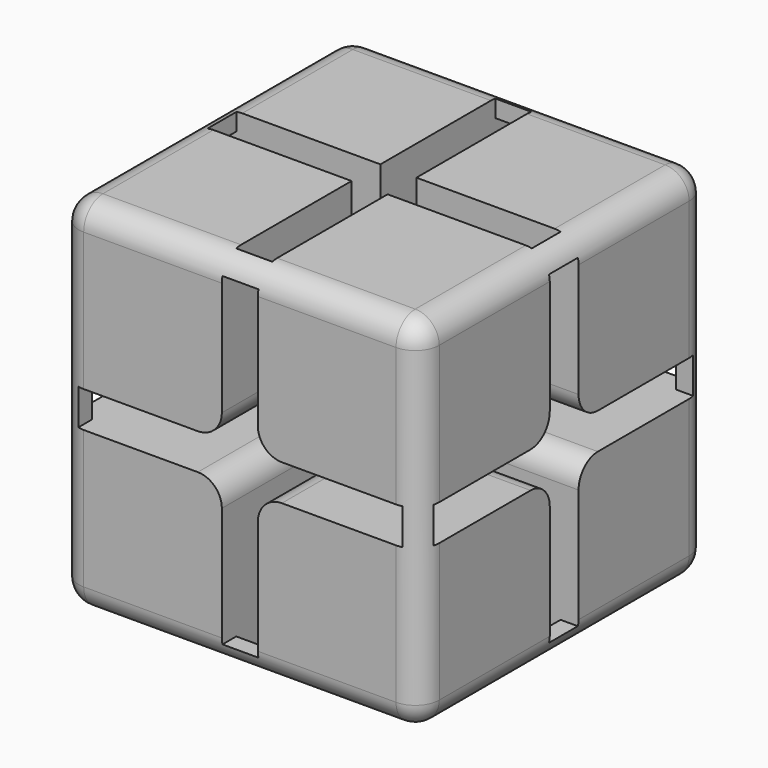
from build123d import *

# Parameters (mm, degrees)
F0_W         = 76.2
F0_H         = 76.2
F1_DEPTH     = 76.2
F3_DEPTH     = 76.2
F5_DEPTH     = 76.2
F7_DEPTH     = 76.2
F8_T1_DEPTH  = 66.04
F8_T3_DEPTH  = 66.04
F8_T5_DEPTH  = 66.04
F8_S9_W      = 5.08
F8_S9_H      = 5.08
F8_T10_DEPTH = 5.08
F8_S15_W     = 5.08
F8_S15_H     = 5.08
F8_T16_DEPTH = 5.08
F8_S21_W     = 5.08
F8_S21_H     = 5.08
F8_T22_DEPTH = 5.08
F8_S27_W     = 5.08
F8_S27_H     = 5.08
F8_T28_DEPTH = 5.08
F8_S33_W     = 5.08
F8_S33_H     = 5.08
F8_T34_DEPTH = 5.08
F8_S39_W     = 5.08
F8_S39_H     = 5.08
F8_T40_DEPTH = 5.08
F8_S45_W     = 5.08
F8_S45_H     = 5.08
F8_T46_DEPTH = 5.08
F8_S51_W     = 5.08
F8_S51_H     = 5.08
F8_T52_DEPTH = 5.08
F9_R         = 5.08


# Not quite as in the source:
# - a fillet or chamfer that OpenCascade refuses, or shapes differently, is made with other operations: its cross-section is extruded or revolved along the edge and cut away or added


with BuildPart() as f1:
    # F0 (on Top) → F1 (new body)
    with BuildSketch(Plane.XY):
        Rectangle(F0_W, F0_H)
    extrude(amount=F1_DEPTH)

    # F2 (on face) → F3 (cut)
    with BuildSketch(Plane.XZ.offset(38.1)):
        Polygon((-3.81, 41.91), (-34.29, 41.91), (-34.29, 34.29), (-3.81, 34.29), (-3.81, 3.81), (3.81, 3.81), (3.81, 34.29), (34.29, 34.29), (34.29, 41.91), (3.81, 41.91), (3.81, 72.39), (-3.81, 72.39), align=None)
    extrude(amount=-F3_DEPTH, mode=Mode.SUBTRACT)

    # F4 (on face) → F5 (cut)
    with BuildSketch(Plane.XY.offset(76.2)):
        Polygon((3.81, 34.29), (-3.81, 34.29), (-3.81, 3.81), (-34.29, 3.81), (-34.29, -3.81), (-3.81, -3.81), (-3.81, -34.29), (3.81, -34.29), (3.81, -3.81), (34.29, -3.81), (34.29, 3.81), (3.81, 3.81), align=None)
    extrude(amount=-F5_DEPTH, mode=Mode.SUBTRACT)

    # F6 (on face) → F7 (cut)
    with BuildSketch(Plane.YZ.offset(38.1)):
        Polygon((-3.81, 41.91), (-34.29, 41.91), (-34.29, 34.29), (-3.81, 34.29), (-3.81, 3.81), (3.81, 3.81), (3.81, 34.29), (34.29, 34.29), (34.29, 41.91), (3.81, 41.91), (3.81, 72.39), (-3.81, 72.39), align=None)
    extrude(amount=-F7_DEPTH, mode=Mode.SUBTRACT)

    # F8: fillet of radius 5.08 on 12 edges, made by hand

    # F8_s2 → F8_t1 (cut)
    with BuildSketch(Plane.XY.offset(5.08)):
        with BuildLine():
            ThreePointArc((33.02, -38.1), (36.6121024484, -36.6121024484), (38.1, -33.02))
            Line((38.1, -33.02), (38.1, -38.1))
            Line((38.1, -38.1), (33.02, -38.1))
        make_face()
        with BuildLine():
            ThreePointArc((-33.02, -38.1), (-36.6121024484, -36.6121024484), (-38.1, -33.02))
            Line((-38.1, -33.02), (-38.1, -38.1))
            Line((-38.1, -38.1), (-33.02, -38.1))
        make_face()
        with BuildLine():
            ThreePointArc((33.02, 38.1), (36.6121024484, 36.6121024484), (38.1, 33.02))
            Line((38.1, 33.02), (38.1, 38.1))
            Line((38.1, 38.1), (33.02, 38.1))
        make_face()
        with BuildLine():
            ThreePointArc((-33.02, 38.1), (-36.6121024484, 36.6121024484), (-38.1, 33.02))
            Line((-38.1, 33.02), (-38.1, 38.1))
            Line((-38.1, 38.1), (-33.02, 38.1))
        make_face()
    extrude(amount=F8_T1_DEPTH, mode=Mode.SUBTRACT)

    # F8_s4 → F8_t3 (cut)
    with BuildSketch(Plane.YZ.offset(-33.02)):
        with BuildLine():
            ThreePointArc((-38.1, 71.12), (-36.6121024484, 74.7121024484), (-33.02, 76.2))
            Line((-33.02, 76.2), (-38.1, 76.2))
            Line((-38.1, 76.2), (-38.1, 71.12))
        make_face()
        with BuildLine():
            ThreePointArc((-38.1, 5.08), (-36.6121024484, 1.4878975516), (-33.02, 0))
            Line((-33.02, 0), (-38.1, 0))
            Line((-38.1, 0), (-38.1, 5.08))
        make_face()
        with BuildLine():
            ThreePointArc((38.1, 71.12), (36.6121024484, 74.7121024484), (33.02, 76.2))
            Line((33.02, 76.2), (38.1, 76.2))
            Line((38.1, 76.2), (38.1, 71.12))
        make_face()
        with BuildLine():
            ThreePointArc((38.1, 5.08), (36.6121024484, 1.4878975516), (33.02, 0))
            Line((33.02, 0), (38.1, 0))
            Line((38.1, 0), (38.1, 5.08))
        make_face()
    extrude(amount=F8_T3_DEPTH, mode=Mode.SUBTRACT)

    # F8_s6 → F8_t5 (cut)
    with BuildSketch(Plane.XZ.offset(-33.02)):
        with BuildLine():
            ThreePointArc((33.02, 76.2), (36.6121024484, 74.7121024484), (38.1, 71.12))
            Line((38.1, 71.12), (38.1, 76.2))
            Line((38.1, 76.2), (33.02, 76.2))
        make_face()
        with BuildLine():
            ThreePointArc((33.02, 0), (36.6121024484, 1.4878975516), (38.1, 5.08))
            Line((38.1, 5.08), (38.1, 0))
            Line((38.1, 0), (33.02, 0))
        make_face()
        with BuildLine():
            ThreePointArc((-38.1, 71.12), (-36.6121024484, 74.7121024484), (-33.02, 76.2))
            Line((-33.02, 76.2), (-38.1, 76.2))
            Line((-38.1, 76.2), (-38.1, 71.12))
        make_face()
        with BuildLine():
            ThreePointArc((-38.1, 5.08), (-36.6121024484, 1.4878975516), (-33.02, 0))
            Line((-33.02, 0), (-38.1, 0))
            Line((-38.1, 0), (-38.1, 5.08))
        make_face()
    extrude(amount=F8_T5_DEPTH, mode=Mode.SUBTRACT)


with BuildPart() as f8_tool8:
    # F8_s9 → F8_t10 (new body)
    with BuildSketch(Plane.XZ.offset(33.02)):
        with Locations((35.56, 2.54)):
            Rectangle(F8_S9_W, F8_S9_H)
    extrude(amount=F8_T10_DEPTH)

    # F8_s11 → F8_t12 (revolve, cut)
    with BuildSketch(Plane(origin=(33.02, -33.02, 5.08), x_dir=(-0.7071067812, 0, 0.7071067812), z_dir=(0.7071067812, 0, 0.7071067812))):
        with BuildLine():
            ThreePointArc((0, -5.08), (5.08, 0), (0, 5.08))
            Line((0, 5.08), (0, -5.08))
        make_face()
    revolve(axis=Axis((33.02, -33.02, 5.08), (0, -1, 0)), mode=Mode.SUBTRACT)


with BuildPart() as f1_1:
    add(f1.part)

    # F8_t7: cut F8_tool8
    add(f8_tool8.part, mode=Mode.SUBTRACT)


with BuildPart() as f8_tool14:
    # F8_s15 → F8_t16 (new body)
    with BuildSketch(Plane.XZ.offset(33.02)):
        with Locations((35.56, 73.66)):
            Rectangle(F8_S15_W, F8_S15_H)
    extrude(amount=F8_T16_DEPTH)

    # F8_s17 → F8_t18 (revolve, cut)
    with BuildSketch(Plane(origin=(33.02, -33.02, 71.12), x_dir=(-0.7071067812, 0, -0.7071067812), z_dir=(-0.7071067812, 0, 0.7071067812))):
        with BuildLine():
            ThreePointArc((0, -5.08), (5.08, 0), (0, 5.08))
            Line((0, 5.08), (0, -5.08))
        make_face()
    revolve(axis=Axis((33.02, -33.02, 71.12), (0, -1, 0)), mode=Mode.SUBTRACT)


with BuildPart() as f1_2:
    add(f1_1.part)

    # F8_t13: cut F8_tool14
    add(f8_tool14.part, mode=Mode.SUBTRACT)


with BuildPart() as f8_tool20:
    # F8_s21 → F8_t22 (new body)
    with BuildSketch(Plane.XZ.offset(33.02)):
        with Locations((-35.56, 73.66)):
            Rectangle(F8_S21_W, F8_S21_H)
    extrude(amount=F8_T22_DEPTH)

    # F8_s23 → F8_t24 (revolve, cut)
    with BuildSketch(Plane(origin=(-33.02, -33.02, 71.12), x_dir=(0.7071067812, 0, -0.7071067812), z_dir=(-0.7071067812, 0, -0.7071067812))):
        with BuildLine():
            ThreePointArc((0, -5.08), (5.08, 0), (0, 5.08))
            Line((0, 5.08), (0, -5.08))
        make_face()
    revolve(axis=Axis((-33.02, -33.02, 71.12), (0, -1, 0)), mode=Mode.SUBTRACT)


with BuildPart() as f1_3:
    add(f1_2.part)

    # F8_t19: cut F8_tool20
    add(f8_tool20.part, mode=Mode.SUBTRACT)


with BuildPart() as f8_tool26:
    # F8_s27 → F8_t28 (new body)
    with BuildSketch(Plane.XZ.offset(-33.02)):
        with Locations((35.56, 73.66)):
            Rectangle(F8_S27_W, F8_S27_H)
    extrude(amount=-F8_T28_DEPTH)

    # F8_s29 → F8_t30 (revolve, cut)
    with BuildSketch(Plane(origin=(33.02, 33.02, 71.12), x_dir=(-0.7071067812, 0, -0.7071067812), z_dir=(0.7071067812, 0, -0.7071067812))):
        with BuildLine():
            ThreePointArc((0, -5.08), (5.08, 0), (0, 5.08))
            Line((0, 5.08), (0, -5.08))
        make_face()
    revolve(axis=Axis((33.02, 33.02, 71.12), (0, 1, 0)), mode=Mode.SUBTRACT)


with BuildPart() as f1_4:
    add(f1_3.part)

    # F8_t25: cut F8_tool26
    add(f8_tool26.part, mode=Mode.SUBTRACT)


with BuildPart() as f8_tool32:
    # F8_s33 → F8_t34 (new body)
    with BuildSketch(Plane.XZ.offset(33.02)):
        with Locations((-35.56, 2.54)):
            Rectangle(F8_S33_W, F8_S33_H)
    extrude(amount=F8_T34_DEPTH)

    # F8_s35 → F8_t36 (revolve, cut)
    with BuildSketch(Plane(origin=(-33.02, -33.02, 5.08), x_dir=(0.7071067812, 0, 0.7071067812), z_dir=(0.7071067812, 0, -0.7071067812))):
        with BuildLine():
            ThreePointArc((0, -5.08), (5.08, 0), (0, 5.08))
            Line((0, 5.08), (0, -5.08))
        make_face()
    revolve(axis=Axis((-33.02, -33.02, 5.08), (0, -1, 0)), mode=Mode.SUBTRACT)


with BuildPart() as f1_5:
    add(f1_4.part)

    # F8_t31: cut F8_tool32
    add(f8_tool32.part, mode=Mode.SUBTRACT)


with BuildPart() as f8_tool38:
    # F8_s39 → F8_t40 (new body)
    with BuildSketch(Plane.XZ.offset(-33.02)):
        with Locations((35.56, 2.54)):
            Rectangle(F8_S39_W, F8_S39_H)
    extrude(amount=-F8_T40_DEPTH)

    # F8_s41 → F8_t42 (revolve, cut)
    with BuildSketch(Plane(origin=(33.02, 33.02, 5.08), x_dir=(-0.7071067812, 0, 0.7071067812), z_dir=(-0.7071067812, 0, -0.7071067812))):
        with BuildLine():
            ThreePointArc((0, -5.08), (5.08, 0), (0, 5.08))
            Line((0, 5.08), (0, -5.08))
        make_face()
    revolve(axis=Axis((33.02, 33.02, 5.08), (0, 1, 0)), mode=Mode.SUBTRACT)


with BuildPart() as f1_6:
    add(f1_5.part)

    # F8_t37: cut F8_tool38
    add(f8_tool38.part, mode=Mode.SUBTRACT)


with BuildPart() as f8_tool44:
    # F8_s45 → F8_t46 (new body)
    with BuildSketch(Plane.XZ.offset(-33.02)):
        with Locations((-35.56, 73.66)):
            Rectangle(F8_S45_W, F8_S45_H)
    extrude(amount=-F8_T46_DEPTH)

    # F8_s47 → F8_t48 (revolve, cut)
    with BuildSketch(Plane(origin=(-33.02, 33.02, 71.12), x_dir=(0.7071067812, 0, -0.7071067812), z_dir=(0.7071067812, 0, 0.7071067812))):
        with BuildLine():
            ThreePointArc((0, -5.08), (5.08, 0), (0, 5.08))
            Line((0, 5.08), (0, -5.08))
        make_face()
    revolve(axis=Axis((-33.02, 33.02, 71.12), (0, 1, 0)), mode=Mode.SUBTRACT)


with BuildPart() as f1_7:
    add(f1_6.part)

    # F8_t43: cut F8_tool44
    add(f8_tool44.part, mode=Mode.SUBTRACT)


with BuildPart() as f8_tool50:
    # F8_s51 → F8_t52 (new body)
    with BuildSketch(Plane.XZ.offset(-33.02)):
        with Locations((-35.56, 2.54)):
            Rectangle(F8_S51_W, F8_S51_H)
    extrude(amount=-F8_T52_DEPTH)

    # F8_s53 → F8_t54 (revolve, cut)
    with BuildSketch(Plane(origin=(-33.02, 33.02, 5.08), x_dir=(0.7071067812, 0, 0.7071067812), z_dir=(-0.7071067812, 0, 0.7071067812))):
        with BuildLine():
            ThreePointArc((0, -5.08), (5.08, 0), (0, 5.08))
            Line((0, 5.08), (0, -5.08))
        make_face()
    revolve(axis=Axis((-33.02, 33.02, 5.08), (0, 1, 0)), mode=Mode.SUBTRACT)


with BuildPart() as f1_8:
    add(f1_7.part)

    # F8_t49: cut F8_tool50
    add(f8_tool50.part, mode=Mode.SUBTRACT)

    # F9
    f9_edges = [f1_8.edges().sort_by_distance(p)[0] for p in [
        (3.81, 20.955, 34.29),
        (3.81, 20.955, 41.91),
        (-3.81, 20.955, 34.29),
        (-3.81, 20.955, 41.91),
        (20.955, 3.81, 34.29),
        (20.955, -3.81, 34.29),
        (20.955, -3.81, 41.91),
        (20.955, 3.81, 41.91),
        (-3.81, -20.955, 34.29),
        (-3.81, -20.955, 41.91),
        (3.81, -20.955, 34.29),
        (3.81, -20.955, 41.91),
        (-20.955, 3.81, 41.91),
        (-20.955, 3.81, 34.29),
        (-20.955, -3.81, 34.29),
        (-20.955, -3.81, 41.91),
    ]]
    fillet(f9_edges, radius=F9_R)


solid = f1_8.part
